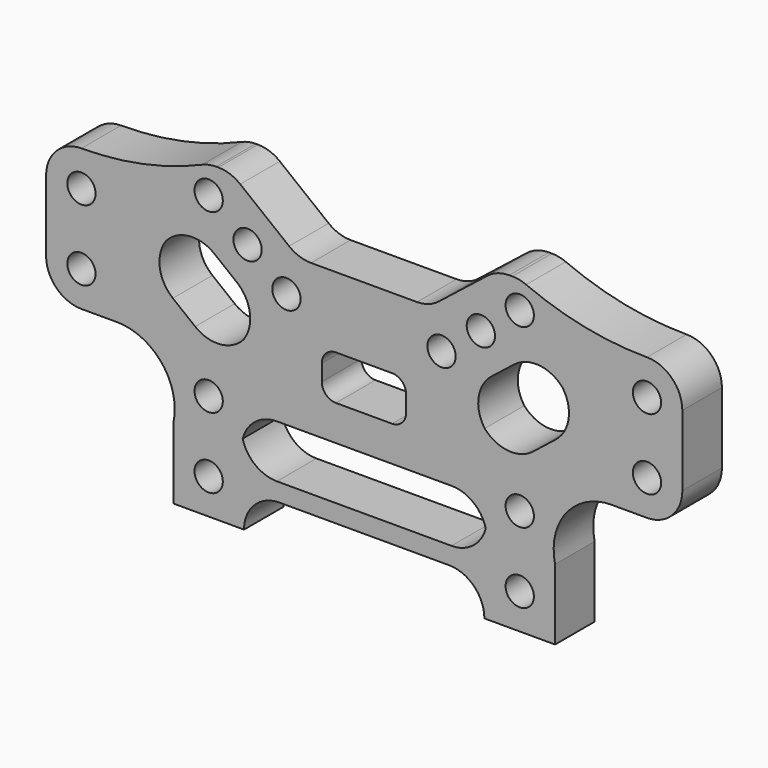
from build123d import *

# Parameters (mm, degrees)
F0_R        = 1
F1_DEPTH    = 3.5
F2_R        = 2.49999
F3_W        = 8.6775156483
F3_H        = 3.7365088891
F4_DEPTH    = 25.4
F5_T1_DEPTH = 3.5
F6_W        = 5.9684215951
F6_H        = 3.1480632909
F7_DEPTH    = 25.4
F8_R        = 1


# Not quite as in the source:
# - a fillet or chamfer that OpenCascade refuses, or shapes differently, is made with other operations: its cross-section is extruded or revolved along the edge and cut away or added
# - a fillet or chamfer is up to 0.001 mm smaller than in the source, because OpenCascade refuses the exact size


with BuildPart() as f1:
    # F0 (on Front) → F1 (new body)
    with BuildSketch(Plane.XZ):
        with BuildLine():
            Line((-13.8224843517, 17.5), (-13.8224843517, 10))
            Line((-13.8224843517, 10), (-13.8224843517, 7.5))
            Line((-13.8224843517, 7.5), (-8.8224843517, 7.5))
            ThreePointArc((-8.8224843517, 7.5), (-5.620922233, 5.961249695), (-4.8224843517, 2.5))
            Line((-4.8224843517, 2.5), (-4.8224843517, 0))
            Line((-4.8224843517, 0), (-4.8224843517, -2.5))
            Line((-4.8224843517, -2.5), (0.1775156483, -2.5))
            Line((0.1775156483, -2.5), (0.1775156483, 0))
            Line((0.1775156483, 0), (8.6775156483, 0))
            Line((8.6775156483, 0), (17.1775156483, 0))
            Line((17.1775156483, 0), (17.1775156483, -2.5))
            Line((17.1775156483, -2.5), (22.1775156483, -2.5))
            Line((22.1775156483, -2.5), (22.1775156483, 0))
            Line((22.1775156483, 0), (22.1775156483, 2.5))
            ThreePointArc((22.1775156483, 2.5), (22.9759535296, 5.961249695), (26.1775156483, 7.5))
            Line((26.1775156483, 7.5), (31.1775156483, 7.5))
            Line((31.1775156483, 7.5), (31.1775156483, 10))
            Line((31.1775156483, 10), (31.1775156483, 17.5))
            Line((31.1775156483, 17.5), (28.6775156483, 17.5))
            ThreePointArc((28.6775156483, 17.5), (24.0740626287, 17.9907408644), (19.6775156483, 19.4409066995))
            Line((19.6775156483, 19.4409066995), (18.069904763, 19.4409066995))
            Line((18.069904763, 19.4409066995), (13.2764897522, 15.6480632909))
            Line((13.2764897522, 15.6480632909), (4.0469631395, 15.6480632909))
            Line((4.0469631395, 15.6480632909), (-0.7712156733, 19.4605013357))
            Line((-0.7712156733, 19.4605013357), (-2.3224843517, 19.4605013357))
            ThreePointArc((-2.3224843517, 19.4605013357), (-6.7169560029, 17.9958056322), (-11.3224843517, 17.5))
            Line((-11.3224843517, 17.5), (-13.8224843517, 17.5))
        make_face()
        with Locations((-2.3224843517, 0)):
            Circle(F0_R, mode=Mode.SUBTRACT)
        with Locations((-2.3224843517, 5)):
            Circle(F0_R, mode=Mode.SUBTRACT)
        with BuildLine():
            ThreePointArc((18.6775156483, 0), (19.6775156483, 1), (20.6775156483, 0))
            ThreePointArc((20.6775156483, 0), (19.6775156483, -1), (18.6775156483, 0))
        make_face(mode=Mode.SUBTRACT)
        with Locations((19.6775156483, 5)):
            Circle(F0_R, mode=Mode.SUBTRACT)
        with BuildLine():
            ThreePointArc((-12.3224843517, 10), (-11.3224843517, 11), (-10.3224843517, 10))
            ThreePointArc((-10.3224843517, 10), (-11.3224843517, 9), (-12.3224843517, 10))
        make_face(mode=Mode.SUBTRACT)
        with Locations((3.1775156483, 13.1480632909)):
            Circle(F0_R, mode=Mode.SUBTRACT)
        with Locations((-11.3224843517, 15)):
            Circle(F0_R, mode=Mode.SUBTRACT)
        with Locations((0.4275156483, 15.3240316454)):
            Circle(F0_R, mode=Mode.SUBTRACT)
        with Locations((-2.3224843517, 17.5)):
            Circle(F0_R, mode=Mode.SUBTRACT)
        with Locations((14.1459372434, 13.1480632909)):
            Circle(F0_R, mode=Mode.SUBTRACT)
        with Locations((28.6775156483, 10)):
            Circle(F0_R, mode=Mode.SUBTRACT)
        with Locations((16.9275156483, 15.3240316454)):
            Circle(F0_R, mode=Mode.SUBTRACT)
        with Locations((19.6775156483, 17.5)):
            Circle(F0_R, mode=Mode.SUBTRACT)
        with Locations((28.6775156483, 15)):
            Circle(F0_R, mode=Mode.SUBTRACT)
    extrude(amount=F1_DEPTH)

    # F2 (radius 2.5 in the source; OpenCascade refuses exactly that, so slightly less here)
    f2_edges = [f1.edges().sort_by_distance(p)[0] for p in [
        (-13.822484, -1.75, 17.5),
        (-13.822484, -1.75, 7.5),
        (31.177516, -1.75, 7.5),
        (31.177516, -1.75, 17.5),
        (-2.322484, -1.75, 19.460501),
        (-0.771216, -1.75, 19.460501),
        (4.046963, -1.75, 15.648063),
        (13.27649, -1.75, 15.648063),
        (18.069905, -1.75, 19.440907),
        (19.677516, -1.75, 19.440907),
        (0.177516, -1.75, 0),
        (17.177516, -1.75, 0),
    ]]
    fillet(f2_edges, radius=F2_R)

    # F3 (on face) → F4 (cut)
    with BuildSketch(Plane.XZ.offset(3.5)):
        Polygon((1.6262469699, 11.1875619551), (-3.8737530301, 15.5394986643), (-6.8168965969, 11.8199386845), (-1.3168965969, 7.4680019754), align=None)
        with Locations((4.3387578242, 3.1317455554)):
            Rectangle(F3_W, F3_H)
        with Locations((13.0162734725, 3.1317455554)):
            Rectangle(F3_W, F3_H)
        Polygon((24.1719278936, 11.8199386845), (21.2287843267, 15.5394986643), (15.7287843267, 11.1875619551), (18.6719278936, 7.4680019754), align=None)
    extrude(amount=-F4_DEPTH, mode=Mode.SUBTRACT)

    # F5: fillet of radius 2.5 on 12 edges, made by hand

    # F5_s2 → F5_t1 (join)
    with BuildSketch(Plane.XZ):
        with BuildLine():
            ThreePointArc((-5.4250217085, 13.5789973285), (-3.7538915599, 14.5109250411), (-1.9132516944, 13.9882299859))
            Line((-1.9132516944, 13.9882299859), (-3.8737530301, 15.5394986643))
            Line((-3.8737530301, 15.5394986643), (-5.4250217085, 13.5789973285))
        make_face()
        with BuildLine():
            ThreePointArc((-5.2656279185, 13.7804400203), (-5.7883229738, 11.9398001548), (-4.8563952612, 10.2686700061))
            Line((-4.8563952612, 10.2686700061), (-6.8168965969, 11.8199386845))
            Line((-6.8168965969, 11.8199386845), (-5.2656279185, 13.7804400203))
        make_face()
        with BuildLine():
            ThreePointArc((-3.2773979327, 9.0192706538), (-1.4367580672, 8.4965755986), (0.2343720815, 9.4285033111))
            Line((0.2343720815, 9.4285033111), (-1.3168965969, 7.4680019754))
            Line((-1.3168965969, 7.4680019754), (-3.2773979327, 9.0192706538))
        make_face()
        with BuildLine():
            ThreePointArc((0.0749782915, 9.2270606194), (0.5976733467, 11.0677004849), (-0.3342543658, 12.7388306335))
            Line((-0.3342543658, 12.7388306335), (1.6262469699, 11.1875619551))
            Line((1.6262469699, 11.1875619551), (0.0749782915, 9.2270606194))
        make_face()
        with BuildLine():
            ThreePointArc((22.2114265578, 10.2686700061), (23.1433542704, 11.9398001548), (22.6206592151, 13.7804400203))
            Line((22.6206592151, 13.7804400203), (24.1719278936, 11.8199386845))
            Line((24.1719278936, 11.8199386845), (22.2114265578, 10.2686700061))
        make_face()
        with BuildLine():
            ThreePointArc((19.268282991, 13.9882299859), (21.1089228565, 14.5109250411), (22.7800530051, 13.5789973285))
            Line((22.7800530051, 13.5789973285), (21.2287843267, 15.5394986643))
            Line((21.2287843267, 15.5394986643), (19.268282991, 13.9882299859))
        make_face()
        with BuildLine():
            ThreePointArc((17.6892856624, 12.7388306335), (16.7573579499, 11.0677004849), (17.2800530051, 9.2270606194))
            Line((17.2800530051, 9.2270606194), (15.7287843267, 11.1875619551))
            Line((15.7287843267, 11.1875619551), (17.6892856624, 12.7388306335))
        make_face()
        with BuildLine():
            ThreePointArc((17.1206592151, 9.4285033111), (18.7917893638, 8.4965755986), (20.6324292293, 9.0192706538))
            Line((20.6324292293, 9.0192706538), (18.6719278936, 7.4680019754))
            Line((18.6719278936, 7.4680019754), (17.1206592151, 9.4285033111))
        make_face()
        with BuildLine():
            ThreePointArc((0, 3.7634911109), (0.732233047, 1.9957241579), (2.5, 1.2634911109))
            Line((2.5, 1.2634911109), (0, 1.2634911109))
            Line((0, 1.2634911109), (0, 3.7634911109))
        make_face()
        with BuildLine():
            ThreePointArc((0, 2.5), (0.732233047, 4.267766953), (2.5, 5))
            Line((2.5, 5), (0, 5))
            Line((0, 5), (0, 2.5))
        make_face()
        with BuildLine():
            ThreePointArc((17.3550312966, 2.5), (16.6227982496, 4.267766953), (14.8550312966, 5))
            Line((14.8550312966, 5), (17.3550312966, 5))
            Line((17.3550312966, 5), (17.3550312966, 2.5))
        make_face()
        with BuildLine():
            ThreePointArc((14.8550312966, 1.2634911109), (16.6227982496, 1.9957241579), (17.3550312966, 3.7634911109))
            Line((17.3550312966, 3.7634911109), (17.3550312966, 1.2634911109))
            Line((17.3550312966, 1.2634911109), (14.8550312966, 1.2634911109))
        make_face()
    extrude(amount=F5_T1_DEPTH)

    # F6 (on face) → F7 (cut)
    with BuildSketch(Plane.XZ.offset(3.5)):
        with Locations((8.6617264459, 9.0740316454)):
            Rectangle(F6_W, F6_H)
    extrude(amount=-F7_DEPTH, mode=Mode.SUBTRACT)

    # F8
    f8_edges = [f1.edges().sort_by_distance(p)[0] for p in [
        (5.677516, -1.75, 7.5),
        (5.677516, -1.75, 10.648063),
        (11.645937, -1.75, 7.5),
        (11.645937, -1.75, 10.648063),
    ]]
    fillet(f8_edges, radius=F8_R)


solid = f1.part
